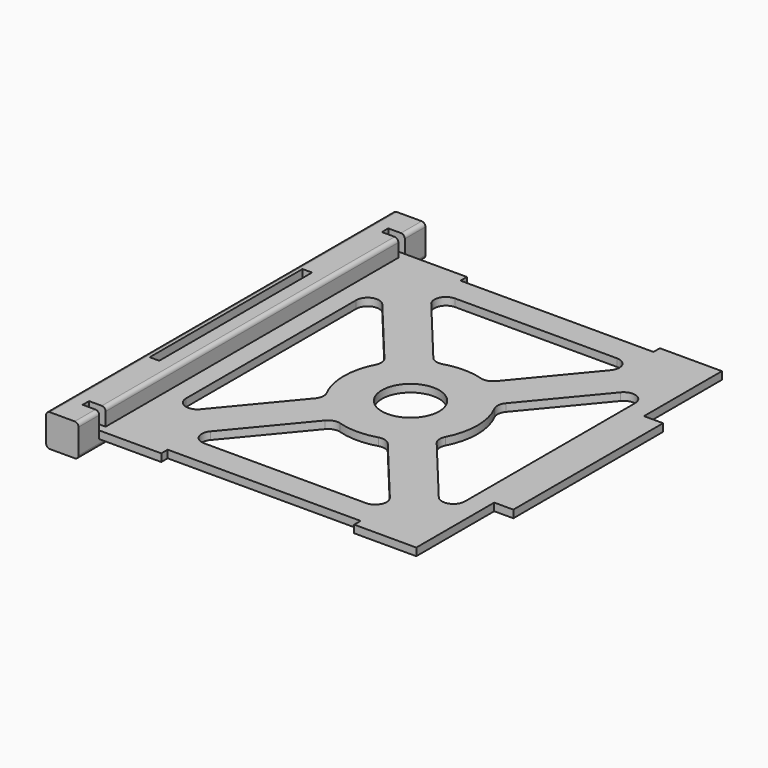
from build123d import *

# Parameters (mm, degrees)
F0_W      = 100
F0_H      = 100
F1_DEPTH  = 2
F2_R      = 7.5
F2_W      = 50.5
F2_H      = 2.1
F3_DEPTH  = 25
F4_W      = 8.5
F4_H      = 100
F4_W_2    = 3.5
F4_H_2    = 49
F5_DEPTH  = 25
F6_W      = 8.5
F6_H      = 8.5
F7_DEPTH  = 56.75
F8_W      = 2.5
F8_H      = 50
F9_DEPTH  = 5.2
F10_R     = 1
F11_W     = 1
F11_H     = 2.1
F11_W_2   = 3.33
F12_DEPTH = 4.5


# Not quite as in the source:
# - a pattern or mirror of a feature is missing from the dataset's text; its kind, count and spacing are read off the source's solid


with BuildPart() as f1:
    # F0 (on Top) → F1 (new body)
    with BuildSketch(Plane.XY):
        Rectangle(F0_W, F0_H)
    extrude(amount=F1_DEPTH)

    # F2 (on face) → F3 (cut)
    with BuildSketch(Plane.XY.offset(2)):
        with BuildLine():
            ThreePointArc((-21.1883002739, 41.0541145875), (-23.9038135596, 39.3292567737), (-23.4967439726, 36.1381063176))
            Line((-23.4967439726, 36.1381063176), (-8.2072148474, 17.7169868897))
            ThreePointArc((-8.2072148474, 17.7169868897), (-6.7654738079, 16.7609181236), (-5.0355363465, 16.7598739167))
            ThreePointArc((-5.0355363465, 16.7598739167), (0, 17.5), (5.0355363465, 16.7598739167))
            ThreePointArc((5.0355363465, 16.7598739167), (6.7654738079, 16.7609181236), (8.2072148474, 17.7169868897))
            Line((8.2072148474, 17.7169868897), (23.4967439726, 36.1381063176))
            ThreePointArc((23.4967439726, 36.1381063176), (23.9038135596, 39.3292567737), (21.1883002739, 41.0541145875))
            Line((21.1883002739, 41.0541145875), (-21.1883002739, 41.0541145875))
        make_face()
        with BuildLine():
            ThreePointArc((-15.5455239175, -8.0365842327), (-17.5, 0), (-15.5455239175, 8.0365842327))
            ThreePointArc((-15.5455239175, 8.0365842327), (-15.2278910436, 9.7371118179), (-15.9020271762, 11.3302926568))
            Line((-15.9020271762, 11.3302926568), (-31.1915563014, 29.7514120847))
            ThreePointArc((-31.1915563014, 29.7514120847), (-34.5184961718, 30.6572233604), (-36.5, 27.8354038148))
            Line((-36.5, 27.8354038148), (-36.5, -27.8354038148))
            ThreePointArc((-36.5, -27.8354038148), (-34.5184961718, -30.6572233604), (-31.1915563014, -29.7514120847))
            Line((-31.1915563014, -29.7514120847), (-15.9020271762, -11.3302926568))
            ThreePointArc((-15.9020271762, -11.3302926568), (-15.2278910436, -9.7371118179), (-15.5455239175, -8.0365842327))
        make_face()
        Circle(F2_R)
        with BuildLine():
            Line((15.9020271762, -11.3302926568), (31.1915563014, -29.7514120847))
            ThreePointArc((31.1915563014, -29.7514120847), (34.5184961718, -30.6572233604), (36.5, -27.8354038148))
            Line((36.5, -27.8354038148), (36.5, 27.8354038148))
            ThreePointArc((36.5, 27.8354038148), (34.5184961718, 30.6572233604), (31.1915563014, 29.7514120847))
            Line((31.1915563014, 29.7514120847), (15.9020271762, 11.3302926568))
            ThreePointArc((15.9020271762, 11.3302926568), (15.2278910436, 9.7371118179), (15.5455239175, 8.0365842327))
            ThreePointArc((15.5455239175, 8.0365842327), (17.5, 0), (15.5455239175, -8.0365842327))
            ThreePointArc((15.5455239175, -8.0365842327), (15.2278910436, -9.7371118179), (15.9020271762, -11.3302926568))
        make_face()
        with BuildLine():
            ThreePointArc((21.1883002739, -41.0541145875), (23.9038135596, -39.3292567737), (23.4967439726, -36.1381063176))
            Line((23.4967439726, -36.1381063176), (8.2072148474, -17.7169868897))
            ThreePointArc((8.2072148474, -17.7169868897), (6.7654738079, -16.7609181236), (5.0355363465, -16.7598739167))
            ThreePointArc((5.0355363465, -16.7598739167), (0, -17.5), (-5.0355363465, -16.7598739167))
            ThreePointArc((-5.0355363465, -16.7598739167), (-6.7654738079, -16.7609181236), (-8.2072148474, -17.7169868897))
            Line((-8.2072148474, -17.7169868897), (-23.4967439726, -36.1381063176))
            ThreePointArc((-23.4967439726, -36.1381063176), (-23.9038135596, -39.3292567737), (-21.1883002739, -41.0541145875))
            Line((-21.1883002739, -41.0541145875), (21.1883002739, -41.0541145875))
        make_face()
        with Locations((0, 48.95)):
            Rectangle(F2_W, F2_H)
        with Locations((0, -48.95)):
            Rectangle(F2_W, F2_H)
    extrude(amount=-F3_DEPTH, mode=Mode.SUBTRACT)

    # F4 (on face) → F5 (cut)
    with BuildSketch(Plane(origin=(0, 0, 0), x_dir=(1, 0, 0), z_dir=(0, 0, -1))):
        with Locations((-45.75, 0)):
            Rectangle(F4_W, F4_H)
        Polygon((50, 50), (41.5, 50), (41.5, 24.5), (46.5, 24.5), (50, 24.5), align=None)
        with Locations((48.25, 0)):
            Rectangle(F4_W_2, F4_H_2)
        Polygon((41.5, -24.5), (41.5, -50), (50, -50), (50, -24.5), (46.5, -24.5), align=None)
    extrude(amount=-F5_DEPTH, mode=Mode.SUBTRACT)

    # F6 (on Front) → F7 (join, symmetric)
    with BuildSketch(Plane.XZ):
        with Locations((-45.75, 2.25)):
            Rectangle(F6_W, F6_H)
    extrude(amount=F7_DEPTH, both=True)

    # F8 (on face) → F9 (cut)
    with BuildSketch(Plane.XY.offset(6.5)):
        with Locations((-47.03, 0)):
            Rectangle(F8_W, F8_H)
    extrude(amount=-F9_DEPTH, mode=Mode.SUBTRACT)

    # F10
    f10_edges = [f1.edges().sort_by_distance(p)[0] for p in [
        (-41.5, 0, -2),
        (-41.5, 0, 6.5),
        (-50, 0, -2),
        (-50, 0, 6.5),
    ]]
    fillet(f10_edges, radius=F10_R)

    # F11 (on face) → F12 (cut, through all)
    with BuildSketch(Plane.XY.offset(6.5)):
        with Locations((-42, 48.95)):
            Rectangle(F11_W, F11_H)
        with Locations((-44.165, 48.95)):
            Rectangle(F11_W_2, F11_H)
    f12 = extrude(amount=-F12_DEPTH, mode=Mode.SUBTRACT)

    # F12_copies: F12 across plane
    add(f12.mirror(Plane(origin=(0, 0, 0), x_dir=(0, 0, -1), z_dir=(0, -1, 0))), mode=Mode.SUBTRACT)


solid = f1.part
